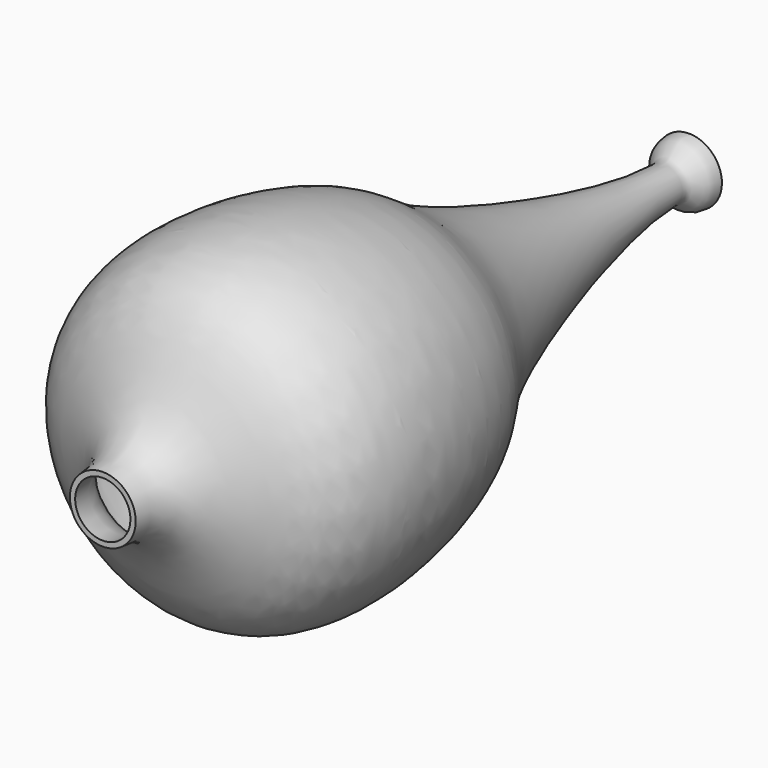
from build123d import *


# Not quite as in the source:
# - the dataset's text gives a spline's control points without its knots; the knots are read off the source's solid


with BuildPart() as f1:
    # F0 (on Right) → F1 (revolve)
    with BuildSketch(Plane.YZ):
        with BuildLine():
            Line((-254, 23.81), (-254, 20))
            add(Edge.make_bspline(
                [(-254, 20), (-203.2, 20), (-204.5033262919, 141.911478125), (-4.9321598974, 107.5987270268), (25.5884560006, 60.8672502828), (203.2, 9.5), (254, 9.5)],
                knots=[0, 0, 0, 0, 0.231974332, 0.498555728, 0.678866593, 1, 1, 1, 1], degree=3))
            add(Edge.make_bspline(
                [(254, 9.5), (266.7, 9.5), (263.8173226654, 20), (276.5173226654, 20)],
                knots=[0, 0, 0, 0, 24.8451166231, 24.8451166231, 24.8451166231, 24.8451166231], degree=3))
            Line((276.5173226654, 20), (276.5173226654, 23.81))
            add(Edge.make_bspline(
                [(254, 13.31), (254.6625, 13.31), (255.8413934342, 13.3785620647), (257.2284819142, 13.6325850704), (258.3162535619, 13.9900919678), (259.2085250215, 14.4290647465), (260.0066701724, 14.9611025853), (260.7849027534, 15.6139446051), (261.5899690012, 16.4055975777), (262.458276617, 17.3331417364), (263.430717001, 18.3743475777), (264.5577035029, 19.4899211676), (265.8941331717, 20.6212588353), (267.4845645206, 21.6888303715), (269.3460885608, 22.6033732178), (271.468636163, 23.2917647579), (273.8396954329, 23.7144995647), (275.5923226654, 23.81), (276.5173226654, 23.81)],
                knots=[0, 0, 0, 0, 0.0625, 0.125, 0.1875, 0.25, 0.3125, 0.375, 0.4375, 0.5, 0.5625, 0.625, 0.6875, 0.75, 0.8125, 0.875, 0.9375, 1, 1, 1, 1], degree=3))
            add(Edge.make_bspline(
                [(-254, 23.81), (-250.7693237287, 23.81), (-244.8076906582, 24.2957513277), (-237.1641042391, 26.2799360823), (-230.5810188827, 29.3538432827), (-224.8251239702, 33.4067791571), (-219.7129964558, 38.3519241491), (-213.5702641703, 45.9934974966), (-208.1986545471, 54.9402448283), (-203.0767660682, 64.5561505106), (-199.2126511401, 71.9362456588), (-195.1722252709, 79.3215943016), (-190.7923153723, 86.548852472), (-186.7164782616, 92.3012534895), (-183.1115514338, 96.6521256708), (-180.2137157134, 99.7656636178), (-177.6192500604, 102.2144843061), (-175.4261434799, 104.0729203361), (-173.1511402585, 105.8589935247), (-170.1758502875, 107.9383603331), (-165.1530516871, 110.9543261837), (-158.4234093809, 114.160315714), (-149.7375063527, 117.1773875659), (-140.5422398991, 119.4332088128), (-127.730424502, 121.5112481326), (-110.9160728923, 122.5159380284), (-90.2105564488, 121.6121913349), (-69.7384232869, 119.0085152402), (-50.2698391462, 115.1017956272), (-32.5752668347, 110.280081836), (-17.4192367752, 104.9196394934), (-5.5167111164, 99.3666091812), (4.2602917838, 93.6057941751), (13.0155333994, 87.6768939909), (20.4540526257, 82.583456522), (27.1278166382, 78.3574798088), (32.6575626781, 75.0943496201), (37.8384529694, 72.2835348063), (42.4057722558, 69.9743598013), (46.0661512321, 68.2083292548), (49.9505889565, 66.4115421261), (55.4118554253, 63.9811887881), (62.7376462863, 60.8886910126), (72.2338630785, 57.1226029207), (85.7137099426, 52.0686289141), (103.8707130454, 45.7654345752), (127.0316525031, 38.4600867355), (150.8503867185, 31.6457678057), (174.6127290262, 25.5538856031), (197.6026196985, 20.4151555956), (219.0987169525, 16.4598335604), (238.3663427755, 13.9160172201), (249.2166319287, 13.31), (254, 13.31)],
                knots=[0, 0, 0, 0, 0.015625, 0.03125, 0.046875, 0.0625, 0.078125, 0.09375, 0.125, 0.140625, 0.15625, 0.171875, 0.1875, 0.203125, 0.2109375, 0.21875, 0.2265625, 0.23046875, 0.234375, 0.2421875, 0.25, 0.265625, 0.28125, 0.296875, 0.3125, 0.34375, 0.375, 0.40625, 0.4375, 0.46875, 0.5, 0.53125, 0.5625, 0.59375, 0.625, 0.640625, 0.65625, 0.671875, 0.6796875, 0.6875, 0.6953125, 0.703125, 0.71875, 0.734375, 0.75, 0.78125, 0.8125, 0.84375, 0.875, 0.90625, 0.9375, 0.96875, 1, 1, 1, 1], degree=3))
        make_face()
    revolve(axis=Axis((0, 0, 0), (0, 1, 0)))


with BuildPart() as f2_1:
    # F2: copy of F1
    add(f1.part)


solid = Compound([f1.part, f2_1.part])
